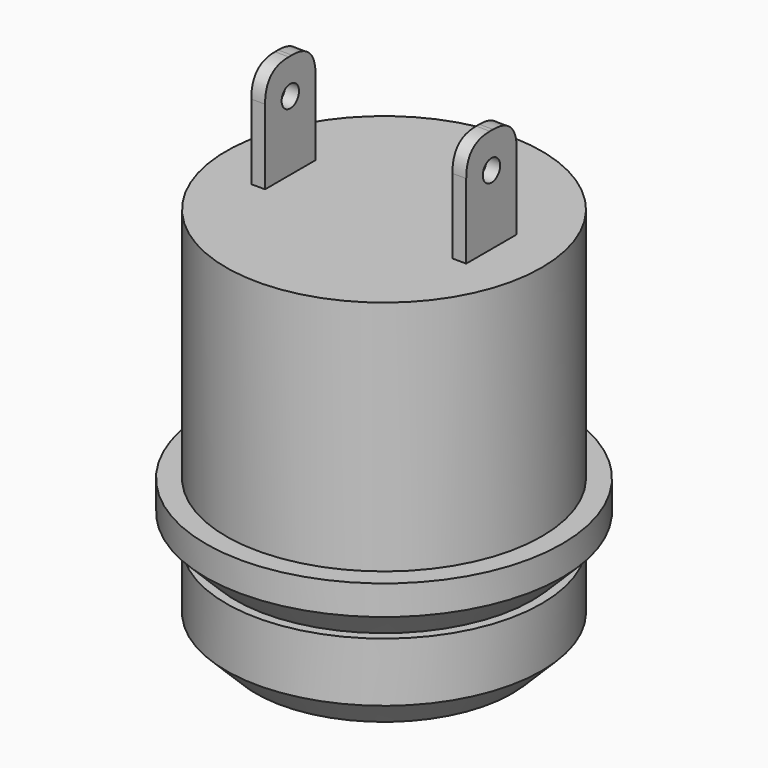
from build123d import *

# Parameters (mm, degrees)
F0_R        = 8
F1_DEPTH    = 15
F0_R_2      = 9.03
F2_DEPTH    = 3
F3_DEPTH    = 4.5
F4_SIZE     = 1.5
F4_2_SIZE   = 1.5
F5_W        = 0.7
F5_H        = 3.2
F6_DEPTH    = 5.3
F7_R        = 0.55
F8_DEPTH    = 25
F9_T1_DEPTH = 8.2
F9_T3_DEPTH = 8.2


# Not quite as in the source:
# - a fillet or chamfer that OpenCascade refuses, or shapes differently, is made with other operations: its cross-section is extruded or revolved along the edge and cut away or added


with BuildPart() as f1:
    # F0 (on Top) → F1 (new body)
    with BuildSketch(Plane.XY):
        Circle(F0_R)
    extrude(amount=F1_DEPTH)

    # F0 (on Top) → F2 (join)
    with BuildSketch(Plane.XY):
        Circle(F0_R_2)
        Circle(F0_R, mode=Mode.SUBTRACT)
        Circle(F0_R)
    extrude(amount=F2_DEPTH)

    # F4#2
    f4_2_edges = [f1.edges().sort_by_distance(p)[0] for p in [
        (-9.03, 0, 0),
    ]]
    chamfer(f4_2_edges, length=F4_2_SIZE)

    # F5 (on face) → F6 (join)
    with BuildSketch(Plane.XY.offset(15)):
        with Locations((-5.1, 0)):
            Rectangle(F5_W, F5_H)
        with Locations((5.1, 0)):
            Rectangle(F5_W, F5_H)
    extrude(amount=F6_DEPTH)

    # F7 (on face) → F8 (cut)
    with BuildSketch(Plane(origin=(-5.45, 0, 0), x_dir=(0, -1, 0), z_dir=(-1, 0, 0))):
        with Locations((0, 18.5127034783)):
            Circle(F7_R)
    extrude(amount=-F8_DEPTH, mode=Mode.SUBTRACT)

    # F9: fillet of radius 1.5 on 4 edges, made by hand

    # F9_s2 → F9_t1 (cut)
    with BuildSketch(Plane.YZ.offset(-9.2)):
        with BuildLine():
            add(Edge.make_bspline(
                [(-1.6, 18.8), (-1.6, 20.3), (-0.1, 20.3)],
                knots=[0, 0, 0, 1, 1, 1], degree=2, weights=[1, 1, 1]))
            Line((-0.1, 20.3), (-1.6, 20.3))
            Line((-1.6, 20.3), (-1.6, 18.8))
        make_face()
        with BuildLine():
            add(Edge.make_bspline(
                [(1.6, 18.8), (1.6, 20.3), (0.1, 20.3)],
                knots=[0, 0, 0, 1, 1, 1], degree=2, weights=[1, 1, 1]))
            Line((0.1, 20.3), (1.6, 20.3))
            Line((1.6, 20.3), (1.6, 18.8))
        make_face()
    extrude(amount=F9_T1_DEPTH, mode=Mode.SUBTRACT)

    # F9_s4 → F9_t3 (cut)
    with BuildSketch(Plane.YZ.offset(1)):
        with BuildLine():
            add(Edge.make_bspline(
                [(-1.6, 18.8), (-1.6, 20.3), (-0.1, 20.3)],
                knots=[0, 0, 0, 1, 1, 1], degree=2, weights=[1, 1, 1]))
            Line((-0.1, 20.3), (-1.6, 20.3))
            Line((-1.6, 20.3), (-1.6, 18.8))
        make_face()
        with BuildLine():
            add(Edge.make_bspline(
                [(1.6, 18.8), (1.6, 20.3), (0.1, 20.3)],
                knots=[0, 0, 0, 1, 1, 1], degree=2, weights=[1, 1, 1]))
            Line((0.1, 20.3), (1.6, 20.3))
            Line((1.6, 20.3), (1.6, 18.8))
        make_face()
    extrude(amount=F9_T3_DEPTH, mode=Mode.SUBTRACT)


with BuildPart() as f3:
    # F0 (on Top) → F3 (new body)
    with BuildSketch(Plane.XY):
        Circle(F0_R)
    extrude(amount=-F3_DEPTH)

    # F4
    f4_edges = [f3.edges().sort_by_distance(p)[0] for p in [
        (-8, 0, -4.5),
    ]]
    chamfer(f4_edges, length=F4_SIZE)


solid = Compound([f1.part, f3.part])
